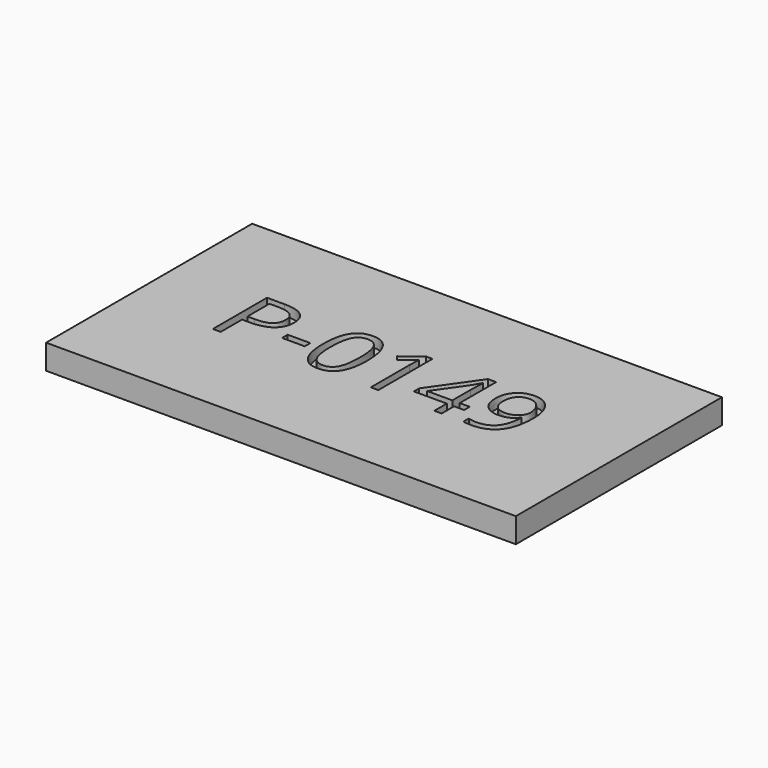
from build123d import *

# Parameters (mm, degrees)
F0_W         = 60.2211547084
F0_H         = 33.0260908231
F1_DEPTH     = 3.175
F2_TEXT_SIZE = 12.146257278
F3_DEPTH     = 1.27


# Not quite as in the source:
# - Text() gives the source's letters only with a copy of the font that has no kerning and outlines rounded to 1/6400 em; it was checked with that copy


with BuildPart() as f1:
    # F0 (on Top) → F1 (new body)
    with BuildSketch(Plane.XY):
        with Locations((23.1480204966, -25.1907450147)):
            Rectangle(F0_W, F0_H)
    extrude(amount=F1_DEPTH)

    # F2 (on face) → F3 (cut)
    with BuildSketch(Plane.XY.offset(3.175)):
        with Locations((3.0313841999, -28.9550255984)):
            Text('P-0149', F2_TEXT_SIZE, font='Open Sans', text_align=(TextAlign.LEFT, TextAlign.BOTTOM))
    extrude(amount=-F3_DEPTH, mode=Mode.SUBTRACT)


solid = f1.part
